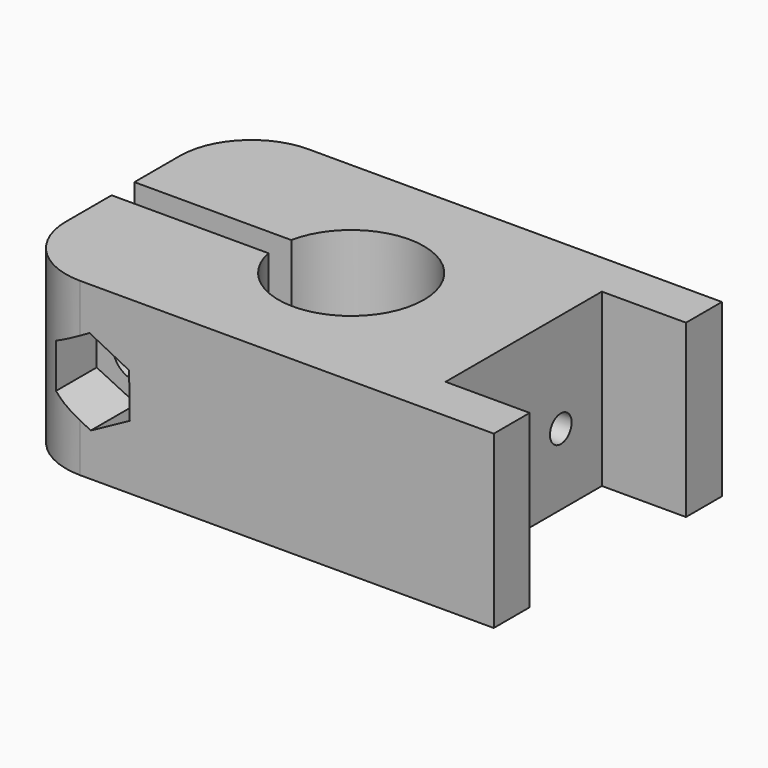
from build123d import *

# Parameters (mm, degrees)
F1_DEPTH     = 12
F2_W         = 5.9
F2_H         = 13.7
F3_DEPTH     = 12.001
F4_R         = 1.6
F5_DEPTH     = 20.001
F6_R         = 0.95
F7_DEPTH     = 7
F9_DEPTH     = 4
F10_R        = 2.8
F11_DEPTH    = 3
F12_T1_DEPTH = 37


# Not quite as in the source:
# - a fillet or chamfer that OpenCascade refuses, or shapes differently, is made with other operations: its cross-section is extruded or revolved along the edge and cut away or added


with BuildPart() as f1:
    # F0 (on Top) → F1 (new body)
    with BuildSketch(Plane.XY):
        with BuildLine():
            Line((18, 10), (-16, 10))
            Line((-16, 10), (-16, 1))
            Line((-16, 1), (-5.0009999, 1))
            ThreePointArc((-5.0009999, 1), (5.1, 0), (-5.0009999, -1))
            Line((-5.0009999, -1), (-16, -1))
            Line((-16, -1), (-16, -10))
            Line((-16, -10), (18, -10))
            Line((18, -10), (18, -6.85))
            Line((18, -6.85), (18, 6.85))
            Line((18, 6.85), (18, 10))
        make_face()
    extrude(amount=F1_DEPTH)

    # F2 (on face) → F3 (cut, through all)
    with BuildSketch(Plane(origin=(0, 0, 0), x_dir=(1, 0, 0), z_dir=(0, 0, -1))):
        with Locations((15.05, 0)):
            Rectangle(F2_W, F2_H)
    extrude(amount=-F3_DEPTH, mode=Mode.SUBTRACT)

    # F4 (on face) → F5 (cut, through all)
    with BuildSketch(Plane.XZ.offset(10)):
        with Locations((-10.3, 6)):
            Circle(F4_R)
    extrude(amount=-F5_DEPTH, mode=Mode.SUBTRACT)

    # F6 (on face) → F7 (cut)
    with BuildSketch(Plane.YZ.offset(12.1)):
        with Locations((-3.25, 5)):
            Circle(F6_R)
        with Locations((3.25, 5)):
            Circle(F6_R)
    extrude(amount=-F7_DEPTH, mode=Mode.SUBTRACT)

    # F8 (on face) → F9 (cut)
    with BuildSketch(Plane.XZ.offset(10)):
        Polygon((-7.5270084947, 4.4889189478), (-7.5736076532, 7.5934053818), (-10.3445898285, 8.994), (-13.0481386516, 7.4672939832), (-13.0481386516, 4.3624578361), (-10.2550660504, 3.006451588), align=None)
    extrude(amount=-F9_DEPTH, mode=Mode.SUBTRACT)

    # F10 (on face) → F11 (cut)
    with BuildSketch(Plane(origin=(0, 10, 0), x_dir=(-1, 0, 0), z_dir=(0, 1, 0))):
        with Locations((10.3, 6)):
            Circle(F10_R)
    extrude(amount=-F11_DEPTH, mode=Mode.SUBTRACT)

    # F12: fillet of radius 5 on 2 edges, made by hand

    # F12_s2 → F12_t1 (cut)
    with BuildSketch(Plane.XY.offset(-12.5)):
        with BuildLine():
            ThreePointArc((-11, -10), (-14.5355339059, -8.5355339059), (-16, -5))
            Line((-16, -5), (-16, -10))
            Line((-16, -10), (-11, -10))
        make_face()
        with BuildLine():
            ThreePointArc((-16, 5), (-14.5355339059, 8.5355339059), (-11, 10))
            Line((-11, 10), (-16, 10))
            Line((-16, 10), (-16, 5))
        make_face()
    extrude(amount=F12_T1_DEPTH, mode=Mode.SUBTRACT)


solid = f1.part
